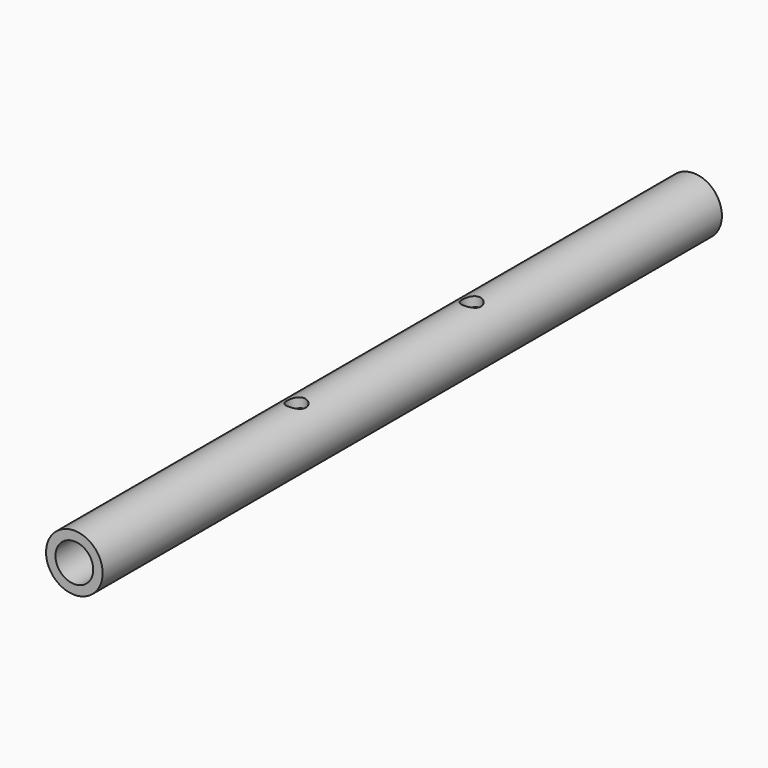
from build123d import *

# Parameters (mm, degrees)
F0_R        = 4.7625
F1_DEPTH    = 130.175
F3_D        = 6.35
F4_W        = 9.525
F4_H        = 9.525
F5_DEPTH    = 130.175
F7_D        = 3.175
F8_T1_DEPTH = 155.575
F11_D       = 3.175


# Not quite as in the source:
# - a fillet or chamfer that OpenCascade refuses, or shapes differently, is made with other operations: its cross-section is extruded or revolved along the edge and cut away or added


with BuildPart() as f1:
    # F0 (on Front) → F1 (new body)
    with BuildSketch(Plane.XZ):
        Circle(F0_R)
    extrude(amount=-F1_DEPTH)

    # F3 (through all)
    with Locations(Plane.XZ):
        with Locations((0, 0)):
            Hole(F3_D / 2)

    # F11 (through all)
    with Locations(Plane.XY.offset(6.604)):
        with Locations((0, 83.5025), (0, 46.6725)):
            Hole(F11_D / 2)


with BuildPart() as f5:
    # F4 (on Front) → F5 (new body)
    with BuildSketch(Plane.XZ):
        with Locations((196.4227657549, 4.7625)):
            Rectangle(F4_W, F4_H)
    extrude(amount=-F5_DEPTH)

    # F7 (through all)
    with Locations(Plane.XY.offset(9.525)):
        with Locations((196.4227657549, 83.5025), (196.4227657549, 46.6725)):
            Hole(F7_D / 2)

    # F8: fillet of radius 5.08 on 4 edges, made by hand

    # F8_s2 → F8_t1 (cut)
    with BuildSketch(Plane.XZ.offset(-142.875)):
        with BuildLine():
            ThreePointArc((196.1052657549, 9.525), (199.6973682033, 8.0371024484), (201.1852657549, 4.445))
            Line((201.1852657549, 4.445), (201.1852657549, 9.525))
            Line((201.1852657549, 9.525), (196.1052657549, 9.525))
        make_face()
        with BuildLine():
            ThreePointArc((191.6602657549, 4.445), (193.1481633065, 8.0371024484), (196.7402657549, 9.525))
            Line((196.7402657549, 9.525), (191.6602657549, 9.525))
            Line((191.6602657549, 9.525), (191.6602657549, 4.445))
        make_face()
        with BuildLine():
            ThreePointArc((196.1052657549, 0), (199.6973682033, 1.4878975516), (201.1852657549, 5.08))
            Line((201.1852657549, 5.08), (201.1852657549, 0))
            Line((201.1852657549, 0), (196.1052657549, 0))
        make_face()
        with BuildLine():
            ThreePointArc((191.6602657549, 5.08), (193.1481633065, 1.4878975516), (196.7402657549, 0))
            Line((196.7402657549, 0), (191.6602657549, 0))
            Line((191.6602657549, 0), (191.6602657549, 5.08))
        make_face()
    extrude(amount=F8_T1_DEPTH, mode=Mode.SUBTRACT)


solid = f1.part
